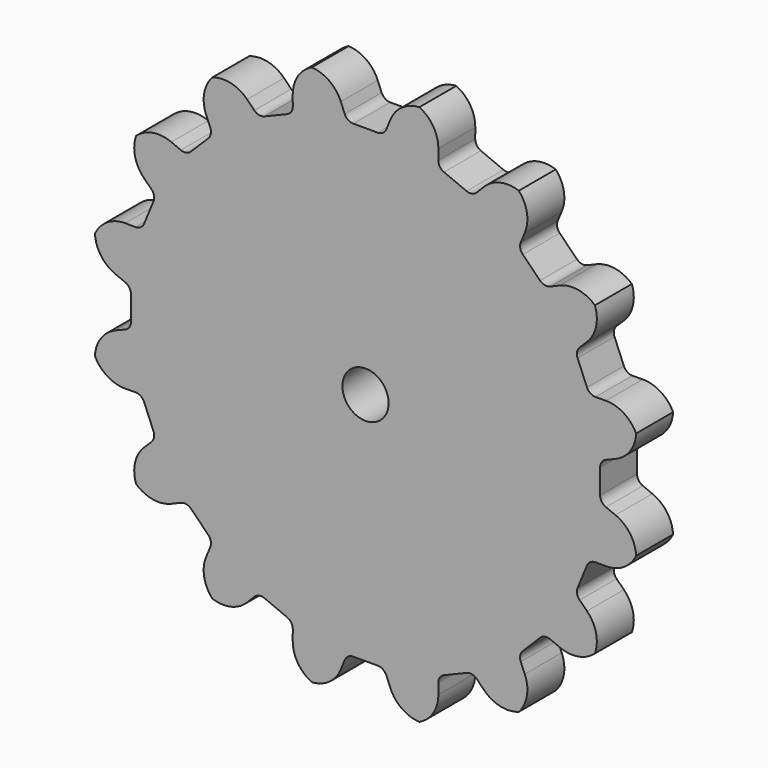
from build123d import *

# Parameters (mm, degrees)
F0_W            = 6.35
F0_H            = 38.1
F3_DEPTH        = 6.35
F3_COPIES_COUNT = 16
F4_T1_DEPTH     = 26.0646341438
F5_R            = 3.175
F6_DEPTH        = 6.35


# Not quite as in the source:
# - a fillet or chamfer that OpenCascade refuses, or shapes differently, is made with other operations: its cross-section is extruded or revolved along the edge and cut away or added
# - a pattern or mirror of a feature is missing from the dataset's text; its kind, count and spacing are read off the source's solid


with BuildPart() as f1:
    # F0 (on Right) → F1 (revolve)
    with BuildSketch(Plane.YZ):
        with Locations((3.175, 57.15)):
            Rectangle(F0_W, F0_H)
    revolve(axis=Axis((0, 3.175, 38.1), (0, 1, 0)))

    # F2 (on Front) → F3 (cut)
    with BuildSketch(Plane.XZ):
        with BuildLine():
            Line((-1.6858047682, 70.3646540642), (0, 70.3646540642))
            Line((0, 70.3646540642), (0, 76.2))
            Line((0, 76.2), (-4.9155252054, 76.2))
            Line((-4.9155252054, 76.2), (-2.862071475, 71.1558047824))
            ThreePointArc((-2.862071475, 71.1558047824), (-2.3945929637, 70.5808422717), (-1.6858047682, 70.3646540642))
        make_face()
        with BuildLine():
            Line((0, 76.2), (0, 70.3646540642))
            Line((0, 70.3646540642), (1.6858047682, 70.3646540642))
            ThreePointArc((1.6858047682, 70.3646540642), (2.3945929637, 70.5808422717), (2.862071475, 71.1558047824))
            Line((2.862071475, 71.1558047824), (4.9155252054, 76.2))
            Line((4.9155252054, 76.2), (0, 76.2))
        make_face()
    f3 = extrude(amount=-F3_DEPTH, mode=Mode.SUBTRACT)

    # F3_copies: F3 ×16 about axis
    f3_copies_axis = Axis((0, 0, 38.1), (0, 1, 0))
    for i in range(1, F3_COPIES_COUNT):
        add(f3.rotate(f3_copies_axis, i * 360 / F3_COPIES_COUNT), mode=Mode.SUBTRACT)

    # F4: fillet of radius 4.572 on 32 edges, made by hand

    # F4_s2 → F4_t1 (cut)
    with BuildSketch(Plane.XZ.offset(-16.2073170719)):
        with BuildLine():
            ThreePointArc((-3.3977215365, 72.4715994549), (-5.5321094799, 74.8088331164), (-8.6730473645, 75.1997068643))
            ThreePointArc((-8.6730473645, 75.1997068643), (-6.7417247933, 75.5987886046), (-4.7923392375, 75.897400501))
            Line((-4.7923392375, 75.897400501), (-3.3977215365, 72.4715994549))
        make_face()
        with BuildLine():
            ThreePointArc((8.6730473645, 75.1997068643), (5.5321094799, 74.8088331164), (3.3977215365, 72.4715994549))
            Line((3.3977215365, 72.4715994549), (4.7923392375, 75.897400501))
            ThreePointArc((4.7923392375, 75.897400501), (6.7417247933, 75.5987886046), (8.6730473645, 75.1997068643))
        make_face()
        with BuildLine():
            ThreePointArc((34.3715994549, 41.4977215365), (36.7088331164, 43.6321094799), (37.0997068643, 46.7730473645))
            ThreePointArc((37.0997068643, 46.7730473645), (37.4987886046, 44.8417247933), (37.797400501, 42.8923392375))
            Line((37.797400501, 42.8923392375), (34.3715994549, 41.4977215365))
        make_face()
        with BuildLine():
            ThreePointArc((37.5946913686, 44.284592218), (36.0315862226, 47.0368595351), (33.0554689758, 48.1143562705))
            Line((33.0554689758, 48.1143562705), (36.7541935335, 48.1368948238))
            ThreePointArc((36.7541935335, 48.1368948238), (37.2243096697, 46.2216235824), (37.5946913686, 44.284592218))
        make_face()
        with BuildLine():
            ThreePointArc((30.4549654962, 54.39252704), (31.7974929347, 57.2588649752), (30.9566282996, 60.3102941071))
            ThreePointArc((30.9566282996, 60.3102941071), (32.0644169018, 58.6787066831), (33.0862958765, 56.9919830926))
            Line((33.0862958765, 56.9919830926), (30.4549654962, 54.39252704))
        make_face()
        with BuildLine():
            ThreePointArc((32.3662249087, 58.2006836988), (29.8688569536, 60.1452726986), (26.7069429938, 60.0018391157))
            Line((26.7069429938, 60.0018391157), (30.1154937781, 61.4381026329))
            ThreePointArc((30.1154937781, 61.4381026329), (31.2827670268, 59.8485283904), (32.3662249087, 58.2006836988))
        make_face()
        with BuildLine():
            ThreePointArc((21.9018391157, 64.8069429938), (22.0452726986, 67.9688569536), (20.1006836988, 70.4662249087))
            ThreePointArc((20.1006836988, 70.4662249087), (21.7485283904, 69.3827670268), (23.3381026329, 68.2154937781))
            Line((23.3381026329, 68.2154937781), (21.9018391157, 64.8069429938))
        make_face()
        with BuildLine():
            ThreePointArc((22.2102941071, 69.0566282996), (19.1588649752, 69.8974929347), (16.29252704, 68.5549654962))
            Line((16.29252704, 68.5549654962), (18.8919830926, 71.1862958765))
            ThreePointArc((18.8919830926, 71.1862958765), (20.5787066831, 70.1644169018), (22.2102941071, 69.0566282996))
        make_face()
        with BuildLine():
            ThreePointArc((10.0143562705, 71.1554689758), (8.9368595351, 74.1315862226), (6.184592218, 75.6946913686))
            ThreePointArc((6.184592218, 75.6946913686), (8.1216235824, 75.3243096697), (10.0368948238, 74.8541935335))
            Line((10.0368948238, 74.8541935335), (10.0143562705, 71.1554689758))
        make_face()
        with BuildLine():
            ThreePointArc((-6.184592218, 75.6946913686), (-8.9368595351, 74.1315862226), (-10.0143562705, 71.1554689758))
            Line((-10.0143562705, 71.1554689758), (-10.0368948238, 74.8541935335))
            ThreePointArc((-10.0368948238, 74.8541935335), (-8.1216235824, 75.3243096697), (-6.184592218, 75.6946913686))
        make_face()
        with BuildLine():
            ThreePointArc((-16.29252704, 68.5549654962), (-19.1588649752, 69.8974929347), (-22.2102941071, 69.0566282996))
            ThreePointArc((-22.2102941071, 69.0566282996), (-20.5787066831, 70.1644169018), (-18.8919830926, 71.1862958765))
            Line((-18.8919830926, 71.1862958765), (-16.29252704, 68.5549654962))
        make_face()
        with BuildLine():
            ThreePointArc((-20.1006836988, 70.4662249087), (-22.0452726986, 67.9688569536), (-21.9018391157, 64.8069429938))
            Line((-21.9018391157, 64.8069429938), (-23.3381026329, 68.2154937781))
            ThreePointArc((-23.3381026329, 68.2154937781), (-21.7485283904, 69.3827670268), (-20.1006836988, 70.4662249087))
        make_face()
        with BuildLine():
            ThreePointArc((-26.7069429938, 60.0018391157), (-29.8688569536, 60.1452726986), (-32.3662249087, 58.2006836988))
            ThreePointArc((-32.3662249087, 58.2006836988), (-31.2827670268, 59.8485283904), (-30.1154937781, 61.4381026329))
            Line((-30.1154937781, 61.4381026329), (-26.7069429938, 60.0018391157))
        make_face()
        with BuildLine():
            ThreePointArc((-30.9566282996, 60.3102941071), (-31.7974929347, 57.2588649752), (-30.4549654962, 54.39252704))
            Line((-30.4549654962, 54.39252704), (-33.0862958765, 56.9919830926))
            ThreePointArc((-33.0862958765, 56.9919830926), (-32.0644169018, 58.6787066831), (-30.9566282996, 60.3102941071))
        make_face()
        with BuildLine():
            ThreePointArc((-33.0554689758, 48.1143562705), (-36.0315862226, 47.0368595351), (-37.5946913686, 44.284592218))
            ThreePointArc((-37.5946913686, 44.284592218), (-37.2243096697, 46.2216235824), (-36.7541935335, 48.1368948238))
            Line((-36.7541935335, 48.1368948238), (-33.0554689758, 48.1143562705))
        make_face()
        with BuildLine():
            ThreePointArc((-37.0997068643, 46.7730473645), (-36.7088331164, 43.6321094799), (-34.3715994549, 41.4977215365))
            Line((-34.3715994549, 41.4977215365), (-37.797400501, 42.8923392375))
            ThreePointArc((-37.797400501, 42.8923392375), (-37.4987886046, 44.8417247933), (-37.0997068643, 46.7730473645))
        make_face()
        with BuildLine():
            ThreePointArc((-34.3715994549, 34.7022784635), (-36.7088331164, 32.5678905201), (-37.0997068643, 29.4269526355))
            ThreePointArc((-37.0997068643, 29.4269526355), (-37.4987886046, 31.3582752067), (-37.797400501, 33.3076607625))
            Line((-37.797400501, 33.3076607625), (-34.3715994549, 34.7022784635))
        make_face()
        with BuildLine():
            ThreePointArc((-37.5946913686, 31.915407782), (-36.0315862226, 29.1631404649), (-33.0554689758, 28.0856437295))
            Line((-33.0554689758, 28.0856437295), (-36.7541935335, 28.0631051762))
            ThreePointArc((-36.7541935335, 28.0631051762), (-37.2243096697, 29.9783764176), (-37.5946913686, 31.915407782))
        make_face()
        with BuildLine():
            ThreePointArc((-30.4549654962, 21.80747296), (-31.7974929347, 18.9411350248), (-30.9566282996, 15.8897058929))
            ThreePointArc((-30.9566282996, 15.8897058929), (-32.0644169018, 17.5212933169), (-33.0862958765, 19.2080169074))
            Line((-33.0862958765, 19.2080169074), (-30.4549654962, 21.80747296))
        make_face()
        with BuildLine():
            ThreePointArc((-32.3662249087, 17.9993163012), (-29.8688569536, 16.0547273014), (-26.7069429938, 16.1981608843))
            Line((-26.7069429938, 16.1981608843), (-30.1154937781, 14.7618973671))
            ThreePointArc((-30.1154937781, 14.7618973671), (-31.2827670268, 16.3514716096), (-32.3662249087, 17.9993163012))
        make_face()
        with BuildLine():
            ThreePointArc((-21.9018391157, 11.3930570062), (-22.0452726986, 8.2311430464), (-20.1006836988, 5.7337750913))
            ThreePointArc((-20.1006836988, 5.7337750913), (-21.7485283904, 6.8172329732), (-23.3381026329, 7.9845062219))
            Line((-23.3381026329, 7.9845062219), (-21.9018391157, 11.3930570062))
        make_face()
        with BuildLine():
            ThreePointArc((-22.2102941071, 7.1433717004), (-19.1588649752, 6.3025070653), (-16.29252704, 7.6450345038))
            Line((-16.29252704, 7.6450345038), (-18.8919830926, 5.0137041235))
            ThreePointArc((-18.8919830926, 5.0137041235), (-20.5787066831, 6.0355830982), (-22.2102941071, 7.1433717004))
        make_face()
        with BuildLine():
            ThreePointArc((-10.0143562705, 5.0445310242), (-8.9368595351, 2.0684137774), (-6.184592218, 0.5053086314))
            ThreePointArc((-6.184592218, 0.5053086314), (-8.1216235824, 0.8756903303), (-10.0368948238, 1.3458064665))
            Line((-10.0368948238, 1.3458064665), (-10.0143562705, 5.0445310242))
        make_face()
        with BuildLine():
            ThreePointArc((-8.6730473645, 1.0002931357), (-5.5321094799, 1.3911668836), (-3.3977215365, 3.7284005451))
            Line((-3.3977215365, 3.7284005451), (-4.7923392375, 0.302599499))
            ThreePointArc((-4.7923392375, 0.302599499), (-6.7417247933, 0.6012113954), (-8.6730473645, 1.0002931357))
        make_face()
        with BuildLine():
            ThreePointArc((3.3977215365, 3.7284005451), (5.5321094799, 1.3911668836), (8.6730473645, 1.0002931357))
            ThreePointArc((8.6730473645, 1.0002931357), (6.7417247933, 0.6012113954), (4.7923392375, 0.302599499))
            Line((4.7923392375, 0.302599499), (3.3977215365, 3.7284005451))
        make_face()
        with BuildLine():
            ThreePointArc((6.184592218, 0.5053086314), (8.9368595351, 2.0684137774), (10.0143562705, 5.0445310242))
            Line((10.0143562705, 5.0445310242), (10.0368948238, 1.3458064665))
            ThreePointArc((10.0368948238, 1.3458064665), (8.1216235824, 0.8756903303), (6.184592218, 0.5053086314))
        make_face()
        with BuildLine():
            ThreePointArc((16.29252704, 7.6450345038), (19.1588649752, 6.3025070653), (22.2102941071, 7.1433717004))
            ThreePointArc((22.2102941071, 7.1433717004), (20.5787066831, 6.0355830982), (18.8919830926, 5.0137041235))
            Line((18.8919830926, 5.0137041235), (16.29252704, 7.6450345038))
        make_face()
        with BuildLine():
            ThreePointArc((20.1006836988, 5.7337750913), (22.0452726986, 8.2311430464), (21.9018391157, 11.3930570062))
            Line((21.9018391157, 11.3930570062), (23.3381026329, 7.9845062219))
            ThreePointArc((23.3381026329, 7.9845062219), (21.7485283904, 6.8172329732), (20.1006836988, 5.7337750913))
        make_face()
        with BuildLine():
            ThreePointArc((26.7069429938, 16.1981608843), (29.8688569536, 16.0547273014), (32.3662249087, 17.9993163012))
            ThreePointArc((32.3662249087, 17.9993163012), (31.2827670268, 16.3514716096), (30.1154937781, 14.7618973671))
            Line((30.1154937781, 14.7618973671), (26.7069429938, 16.1981608843))
        make_face()
        with BuildLine():
            ThreePointArc((30.9566282996, 15.8897058929), (31.7974929347, 18.9411350248), (30.4549654962, 21.80747296))
            Line((30.4549654962, 21.80747296), (33.0862958765, 19.2080169074))
            ThreePointArc((33.0862958765, 19.2080169074), (32.0644169018, 17.5212933169), (30.9566282996, 15.8897058929))
        make_face()
        with BuildLine():
            ThreePointArc((33.0554689758, 28.0856437295), (36.0315862226, 29.1631404649), (37.5946913686, 31.915407782))
            ThreePointArc((37.5946913686, 31.915407782), (37.2243096697, 29.9783764176), (36.7541935335, 28.0631051762))
            Line((36.7541935335, 28.0631051762), (33.0554689758, 28.0856437295))
        make_face()
        with BuildLine():
            ThreePointArc((37.0997068643, 29.4269526355), (36.7088331164, 32.5678905201), (34.3715994549, 34.7022784635))
            Line((34.3715994549, 34.7022784635), (37.797400501, 33.3076607625))
            ThreePointArc((37.797400501, 33.3076607625), (37.4987886046, 31.3582752067), (37.0997068643, 29.4269526355))
        make_face()
    extrude(amount=F4_T1_DEPTH, mode=Mode.SUBTRACT)

    # F5 (on Front) → F6 (cut)
    with BuildSketch(Plane.XZ):
        with Locations((0, 38.1)):
            Circle(F5_R)
    extrude(amount=-F6_DEPTH, mode=Mode.SUBTRACT)


solid = f1.part
